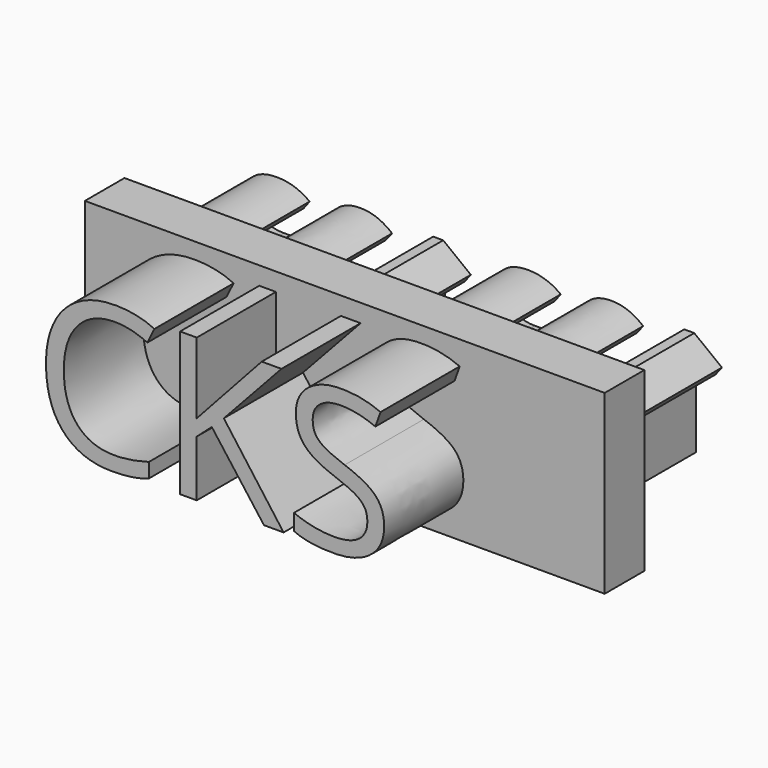
from build123d import *

# Parameters (mm, degrees)
F0_W         = 105.0537899137
F0_H         = 35.742431879
F1_DEPTH     = 10
F2_TEXT_SIZE = 40.5673704032
F3_DEPTH     = 20
F4_TEXT_SIZE = 29.5850435375
F5_DEPTH     = 25


# Not quite as in the source:
# - Text() gives the source's letters only with a copy of the font that has no kerning and outlines rounded to 1/6400 em; it was checked with that copy


with BuildPart() as f1:
    # F0 (on Front) → F1 (new body)
    with BuildSketch(Plane.XZ):
        with Locations((52.5268949568, 17.8712159395)):
            Rectangle(F0_W, F0_H)
    extrude(amount=F1_DEPTH)

    # F2 (on face) → F3 (join)
    with BuildSketch(Plane.XZ.offset(10)):
        with Locations((5.6672631763, 3.1450919341)):
            Text('CKS', F2_TEXT_SIZE, font='Open Sans', text_align=(TextAlign.LEFT, TextAlign.BOTTOM))
    extrude(amount=F3_DEPTH)

    # F4 (on face) → F5 (join)
    with BuildSketch(Plane(origin=(0, 0, 0), x_dir=(-1, 0, 0), z_dir=(0, 1, 0))):
        with Locations((-103.4592762589, 7.8249080107)):
            Text('123123', F4_TEXT_SIZE, font='Open Sans', text_align=(TextAlign.LEFT, TextAlign.BOTTOM))
    extrude(amount=F5_DEPTH)


solid = f1.part
